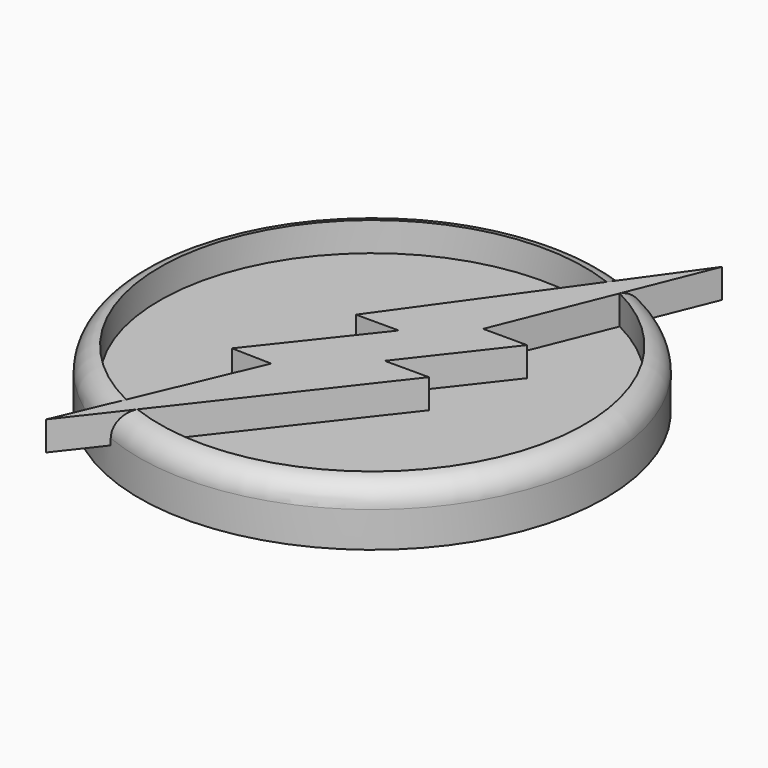
from build123d import *

# Parameters (mm, degrees)
F0_R     = 46.303997109
F1_DEPTH = 6.35
F0_R_2   = 50.7773250867
F2_DEPTH = 12.7
F5_DEPTH = 6.35


# Not quite as in the source:
# - a fillet or chamfer that OpenCascade refuses, or shapes differently, is made with other operations: its cross-section is extruded or revolved along the edge and cut away or added


with BuildPart() as f1:
    # F0 (on Top) → F1 (new body)
    with BuildSketch(Plane.XY):
        Circle(F0_R)
    extrude(amount=F1_DEPTH)

    # F0 (on Top) → F2 (join)
    with BuildSketch(Plane.XY):
        Circle(F0_R_2)
        Circle(F0_R, mode=Mode.SUBTRACT)
    extrude(amount=F2_DEPTH)

    # F3: fillet of radius 5.08 on 1 edges, made by hand

    # F3_s1 → F3_t2 (revolve, cut)
    with BuildSketch(Plane.XZ):
        with BuildLine():
            ThreePointArc((50.7777250867, 7.6554991612), (49.4982109042, 11.0268790536), (46.3040449454, 12.7003971293))
            Line((46.3040449454, 12.7003971293), (46.3648134998, 13.2048869261))
            ThreePointArc((46.3648134998, 13.2048869261), (48.540685016, 13.2081365685), (50.7773250867, 13.2081365685))
            Line((50.7773250867, 13.2081365685), (51.2854616553, 12.7))
            ThreePointArc((51.2854616553, 12.7), (51.2854616553, 10.1777495806), (51.2858616553, 7.6554991612))
            Line((51.2858616553, 7.6554991612), (50.7777250867, 7.6554991612))
        make_face()
    revolve(axis=Axis((0, 0, 12.7), (0, 0, 1)), mode=Mode.SUBTRACT)

    # F4 (on face) → F5 (join)
    with BuildSketch(Plane.XY.offset(6.35)):
        Polygon((-9.3244733289, -15.8572378275), (-26.3735784938, -55.8334334653), (14.7386826575, -3.0078946147), (5.1134219393, -3.0078946147), (20.4086864271, 16.6451374931), (10.8284205198, 16.6451374931), (28.2742083073, 59.8571076989), (-9.3244733289, 7.2189471684), (0, 7.2189471684), (-18.0473700166, -15.6410522759), align=None)
    extrude(amount=F5_DEPTH)


solid = f1.part
